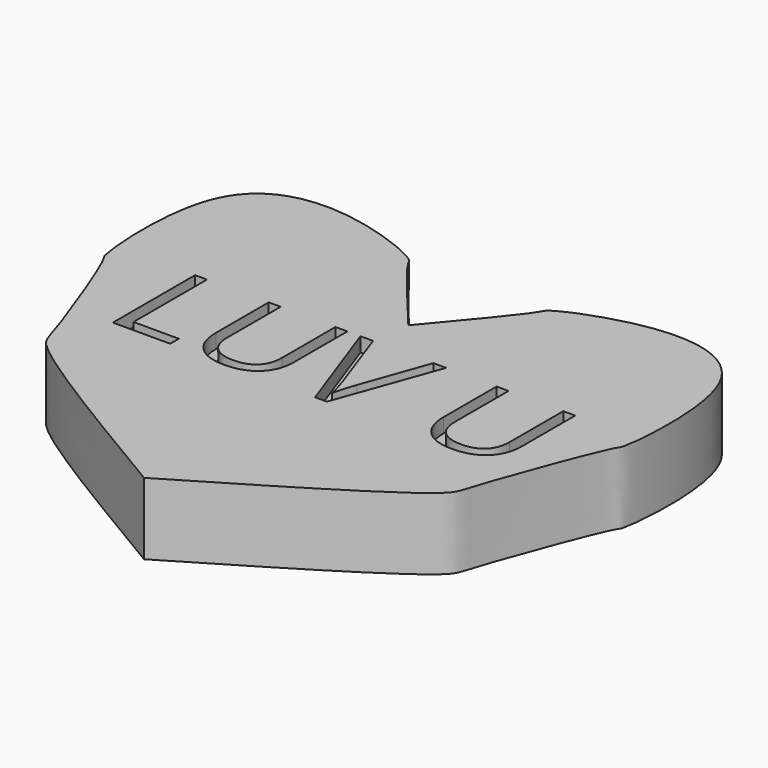
from build123d import *

# Parameters (mm, degrees)
F1_DEPTH     = 12.7
F3_TEXT_SIZE = 25.4999714791
F4_DEPTH     = 2.54


# Not quite as in the source:
# - Text() gives the source's letters only with a copy of the font that has no kerning and outlines rounded to 1/6400 em; it was checked with that copy


with BuildPart() as f1:
    # F0 (on Top) → F1 (new body)
    with BuildSketch(Plane.XY):
        with BuildLine():
            Line((0, -58.5339441895), (0, 0))
            add(Edge.make_bspline(
                [(0, 0), (-5.1001189378, 6.0887934583), (-11.7264763551, 13.9996916523), (-12.0228964649, 15.9832561436), (-28.2681687938, 22.691098623), (-48.7933321408, 18.2946854663), (-46.2692759896, -10.4048631023), (-45.1016375712, -10.2530931414), (-36.6982633629, -32.6578035206), (-36.3930364706, -36.9058101651), (-15.4773612507, -49.3358536772), (0, -58.5339441895)],
                knots=[0, 0, 0, 0, 0.1286770537, 0.1671843656, 0.2869710593, 0.414864426, 0.5601506791, 0.5965686504, 0.7379661374, 0.8060979285, 1, 1, 1, 1], degree=3))
        make_face()
    extrude(amount=F1_DEPTH)

    # F2: F1 across plane


with BuildPart() as f1_1:
    add(f1.part)
    add(f1.part.mirror(Plane.YZ))

    # F3 (on face) → F4 (cut)
    with BuildSketch(Plane.XY.offset(12.7)):
        with Locations((-34.925, -24.9039516357)):
            Text('LUV U', F3_TEXT_SIZE, font='Open Sans', text_align=(TextAlign.LEFT, TextAlign.BOTTOM))
    extrude(amount=-F4_DEPTH, mode=Mode.SUBTRACT)


solid = f1_1.part
